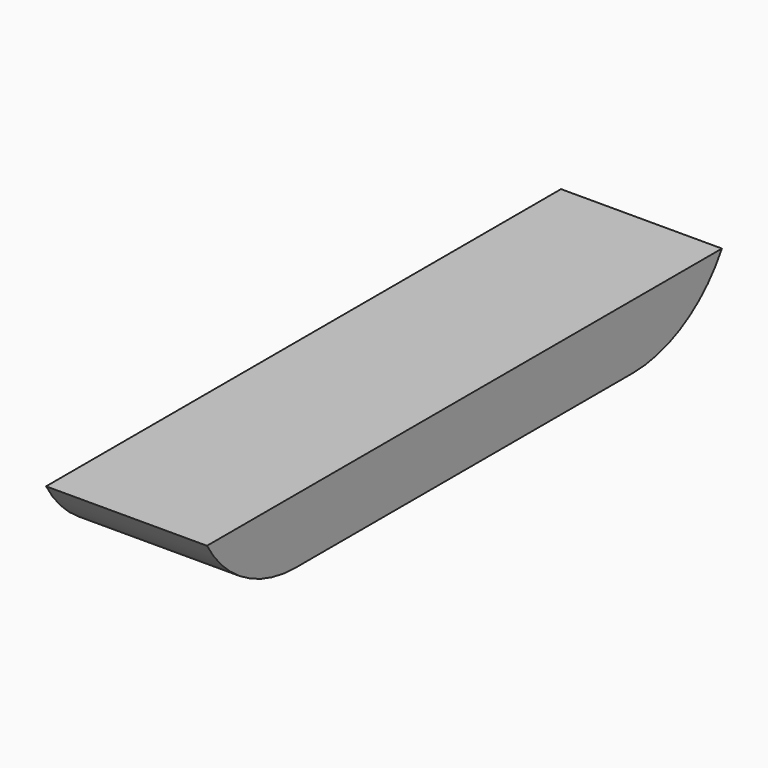
from build123d import *

# Parameters (mm, degrees)
F0_W        = 6.35
F0_H        = 25.4
F1_DEPTH    = 2.54
F2_T1_DEPTH = 28.3470452561


# Not quite as in the source:
# - a fillet or chamfer that OpenCascade refuses, or shapes differently, is made with other operations: its cross-section is extruded or revolved along the edge and cut away or added


with BuildPart() as f1:
    # F0 (on Top) → F1 (new body)
    with BuildSketch(Plane.XY):
        with Locations((-7.7371799469, 21.412451905)):
            Rectangle(F0_W, F0_H)
    extrude(amount=F1_DEPTH)

    # F2: fillet of radius 5.08 on 2 edges, made by hand

    # F2_s2 → F2_t1 (cut)
    with BuildSketch(Plane.YZ.offset(-21.910702575)):
        with BuildLine():
            ThreePointArc((8.712451905, 2.54), (10.5718609562, 0.6805909488), (13.1118609562, 0))
            Line((13.1118609562, 0), (8.712451905, 0))
            Line((8.712451905, 0), (8.712451905, 2.54))
        make_face()
        with BuildLine():
            ThreePointArc((34.112451905, 2.54), (32.2530428538, 0.6805909488), (29.7130428538, 0))
            Line((29.7130428538, 0), (34.112451905, 0))
            Line((34.112451905, 0), (34.112451905, 2.54))
        make_face()
    extrude(amount=F2_T1_DEPTH, mode=Mode.SUBTRACT)


solid = f1.part
